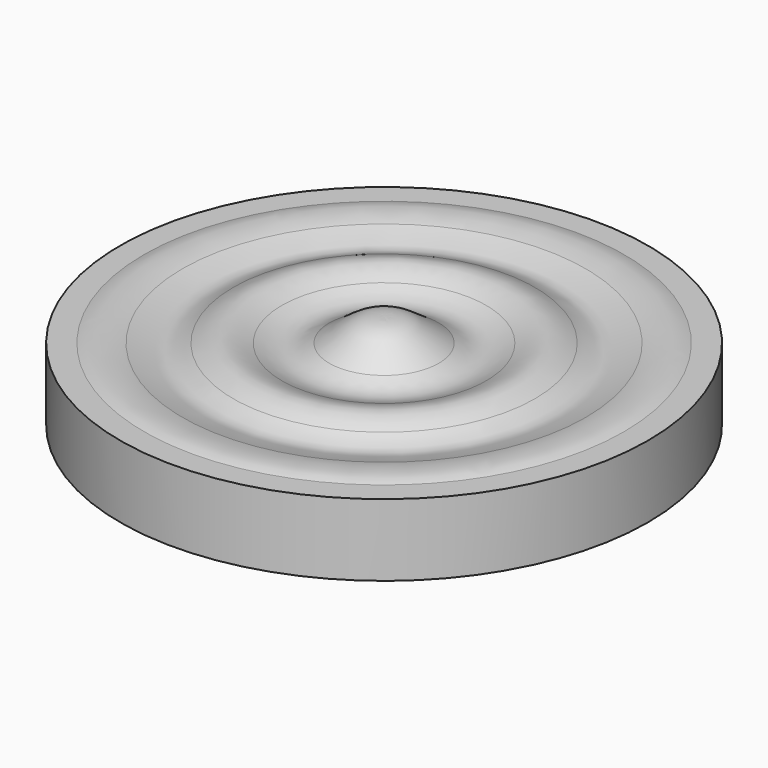
from build123d import *

# Parameters (mm, degrees)
F0_R     = 11
F1_DEPTH = 3
F2_R     = 10
F3_DEPTH = 2


with BuildPart() as f1:
    # F0 (on Top) → F1 (new body)
    with BuildSketch(Plane.XY):
        Circle(F0_R)
    extrude(amount=F1_DEPTH)

    # F2 (on face) → F3 (cut)
    with BuildSketch(Plane.XY.offset(3)):
        Circle(F2_R)
    extrude(amount=-F3_DEPTH, mode=Mode.SUBTRACT)

    # F4 (on Front) → F5 (revolve)
    with BuildSketch(Plane.XZ):
        with BuildLine():
            add(Edge.make_bspline(
                [(-10, 3), (-9.5631365163, 3.1947120998), (-8.9358639257, 3.1521992443), (-8.3988746628, 3)],
                knots=[0, 0, 0, 0, 0.1598537325, 0.1598537325, 0.1598537325, 0.1598537325], degree=3))
            Line((-10, 3), (-8.3988746628, 3))
        make_face()
        with BuildLine():
            Line((-8.3988746628, 3), (-10, 3))
            Line((-10, 3), (-10, 2.2))
            Line((-10, 2.2), (0, 2.2))
            Line((0, 2.2), (0, 3))
            Line((0, 3), (-2.2816949674, 3))
            add(Edge.make_bspline(
                [(-4.2584559222, 3), (-3.9238062504, 2.8445189646), (-3.2540976505, 2.5415343681), (-2.5906789659, 2.8182773792), (-2.2816949674, 3)],
                knots=[0.5757910273, 0.5757910273, 0.5757910273, 0.5757910273, 0.6661755998, 0.754812685, 0.754812685, 0.754812685, 0.754812685], degree=3))
            Line((-4.2584559222, 3), (-6.2872854841, 3))
            add(Edge.make_bspline(
                [(-8.3988746628, 3), (-7.8910468525, 2.8560660067), (-7.2552687251, 2.4957672366), (-6.5324171697, 2.8740056535), (-6.2872854841, 3)],
                knots=[0.1598537325, 0.1598537325, 0.1598537325, 0.1598537325, 0.3110265335, 0.3848969639, 0.3848969639, 0.3848969639, 0.3848969639], degree=3))
        make_face()
        with BuildLine():
            add(Edge.make_bspline(
                [(-6.2872854841, 3), (-5.9671465556, 3.1645470474), (-5.3071713867, 3.4963401186), (-4.6080475442, 3.1624231904), (-4.2584559222, 3)],
                knots=[0.3848969639, 0.3848969639, 0.3848969639, 0.3848969639, 0.4813708261, 0.5757910273, 0.5757910273, 0.5757910273, 0.5757910273], degree=3))
            Line((-6.2872854841, 3), (-4.2584559222, 3))
        make_face()
        with BuildLine():
            Line((-2.2816949674, 3), (0, 3))
            Line((0, 3), (0, 4))
            add(Edge.make_bspline(
                [(-2.2816949674, 3), (-1.9564930944, 3.191260832), (-1.1585189995, 3.8240848781), (-0.654182455, 4.0144366212), (0, 4)],
                knots=[0.754812685, 0.754812685, 0.754812685, 0.754812685, 0.8481021313, 1, 1, 1, 1], degree=3))
        make_face()
    revolve(axis=Axis((0, 0, 3.1), (0, 0, 1)))


solid = f1.part
